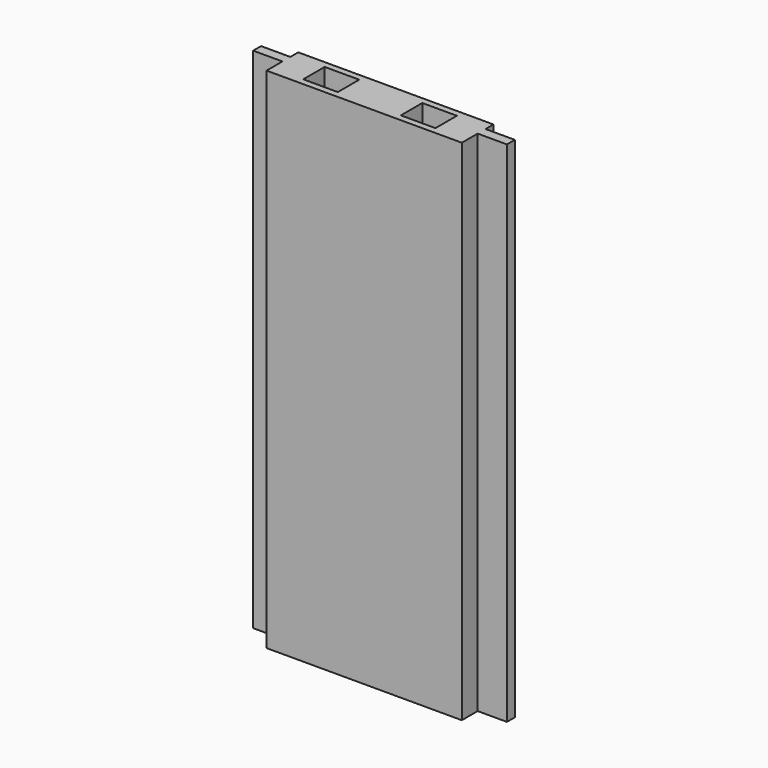
from build123d import *

# Parameters (mm, degrees)
F0_W     = 2.2499504322
F0_H     = 1.7434554408
F1_DEPTH = 1.1348915286
F3_DEPTH = 1.8342579715
F4_DEPTH = 33.0712201539


# Not quite as in the source:
# - the program builds the solid bodies; features that only make, move or delete a surface that nothing else refers to are left out


with BuildPart() as f1:
    # F0 (on Top) → F1 (new body)
    with BuildSketch(Plane.XY):
        Polygon((6.35, 1.2873262627), (-6.35, 1.2873262627), (-6.35, 0.6436631313), (-8.2549656289, 0.6436631313), (-8.2549656289, 0), (-6.35, 0), (-6.35, -1.2873262627), (6.35, -1.2873262627), (6.35, 0), (8.2549656289, 0), (8.2549656289, 0.6436631313), (6.35, 0.6436631313), align=None)
        with Locations((3.175, 0)):
            Rectangle(F0_W, F0_H, mode=Mode.SUBTRACT)
        with Locations((-3.175, 0)):
            Rectangle(F0_W, F0_H, mode=Mode.SUBTRACT)
    extrude(amount=F1_DEPTH)

    # F0 (on Top) → F3 (join)
    with BuildSketch(Plane.XY):
        with Locations((-3.175, 0)):
            Rectangle(F0_W, F0_H)
    extrude(amount=F3_DEPTH)

    # F0 (on Top) → F4 (join)
    with BuildSketch(Plane.XY):
        Polygon((6.35, 1.2873262627), (-6.35, 1.2873262627), (-6.35, 0.6436631313), (-8.2549656289, 0.6436631313), (-8.2549656289, 0), (-6.35, 0), (-6.35, -1.2873262627), (6.35, -1.2873262627), (6.35, 0), (8.2549656289, 0), (8.2549656289, 0.6436631313), (6.35, 0.6436631313), align=None)
        with Locations((3.175, 0)):
            Rectangle(F0_W, F0_H, mode=Mode.SUBTRACT)
        with Locations((-3.175, 0)):
            Rectangle(F0_W, F0_H, mode=Mode.SUBTRACT)
    extrude(amount=F4_DEPTH)


solid = f1.part
